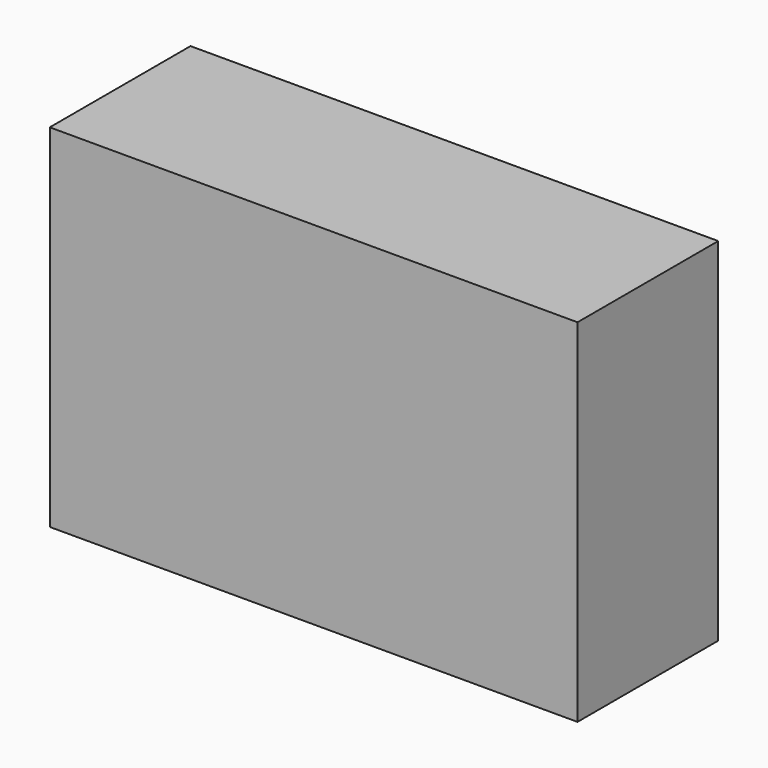
from build123d import *

# Parameters (mm, degrees)
F2_DEPTH = 25.4


# Not quite as in the source:
# - the program builds the solid bodies; features that only make, move or delete a surface that nothing else refers to are left out


with BuildPart() as f2:
    # F0 (on Front) → F2 (new body)
    with BuildSketch(Plane.XZ):
        with BuildLine():
            ThreePointArc((2.63e-08, -25.4), (17.9605122514, -17.9605122328), (25.4, 0))
            ThreePointArc((25.4, 0), (17.9605122427, 17.9605122416), (1.5e-09, 25.4))
            ThreePointArc((1.5e-09, 25.4), (-25.4, -1.24e-08), (2.63e-08, -25.4))
        make_face()
        with BuildLine():
            ThreePointArc((1.5e-09, 25.4), (17.9605122427, 17.9605122416), (25.4, 0))
            ThreePointArc((25.4, 0), (17.9605122514, -17.9605122328), (2.63e-08, -25.4))
            Line((2.63e-08, -25.4), (38.1, -25.4))
            Line((38.1, -25.4), (38.1, 25.4))
            Line((38.1, 25.4), (1.5e-09, 25.4))
        make_face()
        with BuildLine():
            ThreePointArc((2.63e-08, -25.4), (-25.4, -1.24e-08), (1.5e-09, 25.4))
            Line((1.5e-09, 25.4), (-38.1, 25.4))
            Line((-38.1, 25.4), (-38.1, -25.4))
            Line((-38.1, -25.4), (2.63e-08, -25.4))
        make_face()
    extrude(amount=F2_DEPTH)


solid = f2.part
